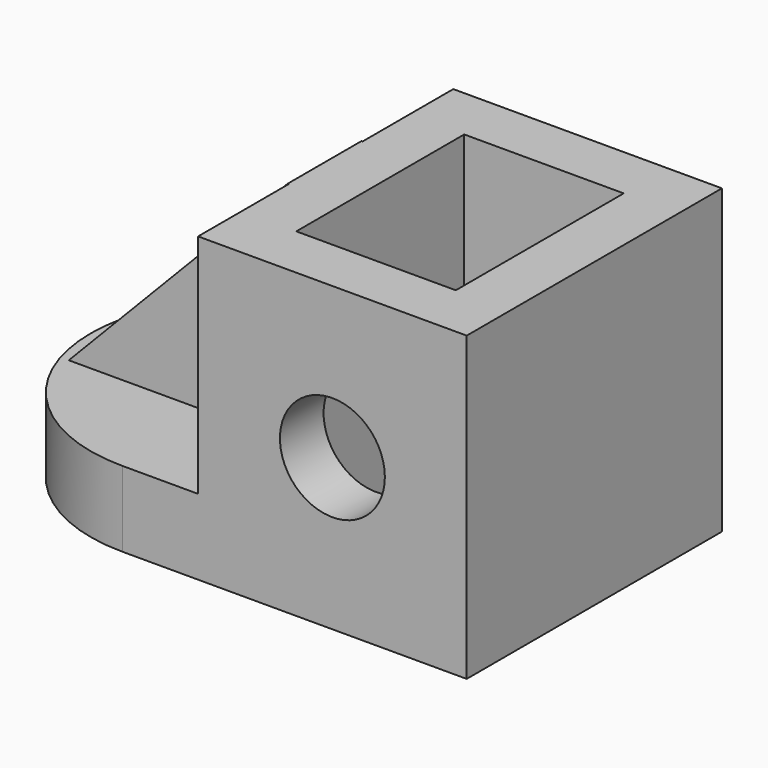
from build123d import *

# Parameters (mm, degrees)
F0_W     = 1422.4
F0_H     = 457.2
F0_R     = 317.5
F1_DEPTH = 1930.4
F2_R     = 965.19999
F4_DEPTH = 1330.96
F5_SIZE2 = 1324.538714
F5_SIZE  = 1371.59999
F6_W     = 965.2
F6_H     = 1270
F7_DEPTH = 4841.24


# Not quite as in the source:
# - a fillet or chamfer is up to 0.001 mm smaller than in the source, because OpenCascade refuses the exact size


with BuildPart() as f1:
    # F0 (on Front) → F1 (new body)
    with BuildSketch(Plane.XZ):
        with Locations((711.2, 228.6)):
            Rectangle(F0_W, F0_H)
        Polygon((1422.4, 457.2), (1422.4, 0), (3048, 0), (3048, 1828.8), (1422.4, 1828.8), align=None)
        with Locations((2235.2, 914.4)):
            Circle(F0_R, mode=Mode.SUBTRACT)
    extrude(amount=F1_DEPTH)

    # F2 (radius 965.2 in the source; OpenCascade refuses exactly that, so slightly less here)
    f2_edges = [f1.edges().sort_by_distance(p)[0] for p in [
        (0, 0, 228.6),
        (0, -1930.4, 228.6),
    ]]
    fillet(f2_edges, radius=F2_R)

    # F3 (on face) → F4 (join)
    with BuildSketch(Plane(origin=(1422.4, 0, 0), x_dir=(0, -1, 0), z_dir=(-1, 0, 0))):
        Polygon((1244.6, 1354.5855283737), (1244.6, 1828.8), (685.8, 1828.8), (685.8, 457.2), (1244.6, 457.2), align=None)
    extrude(amount=F4_DEPTH)

    # F5 (size 1371.6 and 1324.5387235254 in the source; OpenCascade refuses exactly that, so slightly less here)
    f5_edges = [f1.edges().sort_by_distance(p)[0] for p in [
        (91.44, -965.2, 1828.8),
    ]]
    f5_side = f1.faces().sort_by_distance((91.44, -965.2, 1143))[0]
    chamfer(f5_edges, length=F5_SIZE, length2=F5_SIZE2, reference=f5_side)

    # F6 (on face) → F7 (cut)
    with BuildSketch(Plane.XY.offset(1828.8)):
        with Locations((2235.2, -965.2)):
            Rectangle(F6_W, F6_H)
    extrude(amount=-F7_DEPTH, mode=Mode.SUBTRACT)


solid = f1.part
